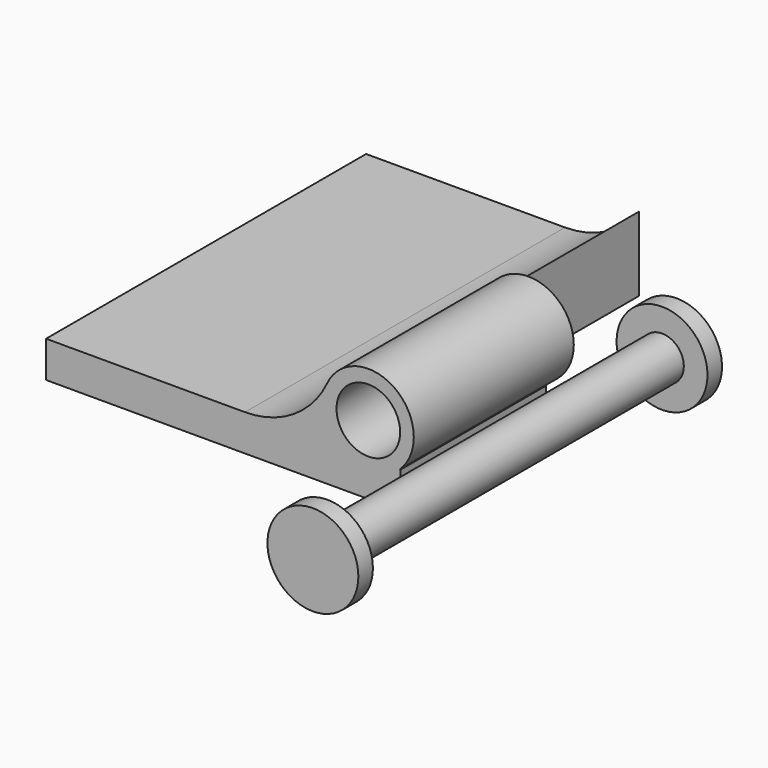
from build123d import *

# Parameters (mm, degrees)
F0_W         = 4.5
F0_H         = 10
F1_DEPTH     = 2
F2_R         = 2.5
F2_R_2       = 1.75
F3_DEPTH     = 11
F4_T4_DEPTH  = 22.646276463
F4_T11_DEPTH = 22.646276463
F4_T18_DEPTH = 10
F4_T23_DEPTH = 10
F5_R         = 1.2
F6_DEPTH     = 11.5
F7_R         = 2.5
F8_DEPTH     = 1
F9_R         = 2.5
F10_DEPTH    = 1


# Not quite as in the source:
# - a fillet or chamfer that OpenCascade refuses, or shapes differently, is made with other operations: its cross-section is extruded or revolved along the edge and cut away or added


with BuildPart() as f1:
    # F0 (on Top) → F1 (new body)
    with BuildSketch(Plane.XY):
        Polygon((-15, 0), (0, 0), (0, 10), (0, 22), (-15, 22), align=None)
        with Locations((2.25, 5)):
            Rectangle(F0_W, F0_H)
    extrude(amount=F1_DEPTH)

    # F2 (on Front) → F3 (join)
    with BuildSketch(Plane.XZ):
        with Locations((2.7228465769, 3.8068606518)):
            Circle(F2_R)
        with Locations((2.7228465769, 3.8068606518)):
            Circle(F2_R_2, mode=Mode.SUBTRACT)
    extrude(amount=-F3_DEPTH)

    # F4: fillet of radius 5 on 1 edges, made by hand


with BuildPart() as f4_tool2:
    # F4_s3 → F4_t4 (new body)
    with BuildSketch(Plane.XZ.offset(-22.646276463)):
        with BuildLine():
            ThreePointArc((-4.0634529377, 2), (-1.3842550939, 2.7784009056), (0.4607467387, 4.8712404345))
            ThreePointArc((0.4607467387, 4.8712404345), (0.2650409494, 3.3494860821), (0.9950576474, 2))
            Line((0.9950576474, 2), (-4.0634529377, 2))
        make_face()
    extrude(amount=F4_T4_DEPTH)

    split(bisect_by=Plane.XZ.offset(-22), keep=Keep.TOP)

    split(bisect_by=Plane.YZ, keep=Keep.BOTTOM)

    split(bisect_by=Plane.XZ.offset(-11), keep=Keep.BOTTOM)


with BuildPart() as f1_1:
    add(f1.part)

    # F4_t1: union F4_tool2
    add(f4_tool2.part)


with BuildPart() as f4_tool9:
    # F4_s10 → F4_t11 (new body)
    with BuildSketch(Plane.XZ.offset(-22.646276463)):
        with BuildLine():
            ThreePointArc((-4.0634529377, 2), (-1.3842550939, 2.7784009056), (0.4607467387, 4.8712404345))
            ThreePointArc((0.4607467387, 4.8712404345), (0.2650409494, 3.3494860821), (0.9950576474, 2))
            Line((0.9950576474, 2), (-4.0634529377, 2))
        make_face()
    extrude(amount=F4_T11_DEPTH)

    split(bisect_by=Plane.YZ, keep=Keep.BOTTOM)

    split(bisect_by=Plane.XZ.offset(-10), keep=Keep.BOTTOM)

    split(bisect_by=Plane.XZ.offset(-11), keep=Keep.TOP)


with BuildPart() as f1_2:
    add(f1_1.part)

    # F4_t8: union F4_tool9
    add(f4_tool9.part)


with BuildPart() as f4_tool16:
    # F4_s17 → F4_t18 (new body)
    with BuildSketch(Plane.XZ.offset(-10)):
        with BuildLine():
            ThreePointArc((-4.0634529377, 2), (-1.3842550939, 2.7784009056), (0.4607467387, 4.8712404345))
            ThreePointArc((0.4607467387, 4.8712404345), (0.2650409494, 3.3494860821), (0.9950576474, 2))
            Line((0.9950576474, 2), (-4.0634529377, 2))
        make_face()
    extrude(amount=F4_T18_DEPTH)

    split(bisect_by=Plane.YZ, keep=Keep.BOTTOM)


with BuildPart() as f1_3:
    add(f1_2.part)

    # F4_t15: union F4_tool16
    add(f4_tool16.part)


with BuildPart() as f4_tool21:
    # F4_s22 → F4_t23 (new body)
    with BuildSketch(Plane.XZ.offset(-10)):
        with BuildLine():
            ThreePointArc((-4.0634529377, 2), (-1.3842550939, 2.7784009056), (0.4607467387, 4.8712404345))
            ThreePointArc((0.4607467387, 4.8712404345), (0.2650409494, 3.3494860821), (0.9950576474, 2))
            Line((0.9950576474, 2), (-4.0634529377, 2))
        make_face()
    extrude(amount=F4_T23_DEPTH)

    split(bisect_by=Plane.YZ, keep=Keep.TOP)


with BuildPart() as f1_4:
    add(f1_3.part)

    # F4_t20: union F4_tool21
    add(f4_tool21.part)


with BuildPart() as f6:
    # F5 (on Front) → F6 (new body, symmetric)
    with BuildSketch(Plane.XZ):
        with Locations((9.6738887951, 4.4031692669)):
            Circle(F5_R)
    extrude(amount=F6_DEPTH, both=True)

    # F7 (on face) → F8 (join)
    with BuildSketch(Plane(origin=(0, 11.5, 0), x_dir=(-1, 0, 0), z_dir=(0, 1, 0))):
        with Locations((-9.6738887951, 4.4031692669)):
            Circle(F7_R)
    extrude(amount=F8_DEPTH)

    # F9 (on face) → F10 (join)
    with BuildSketch(Plane.XZ.offset(11.5)):
        with Locations((9.6738887951, 4.4031692669)):
            Circle(F9_R)
    extrude(amount=F10_DEPTH)


solid = Compound([f1_4.part, f6.part])
